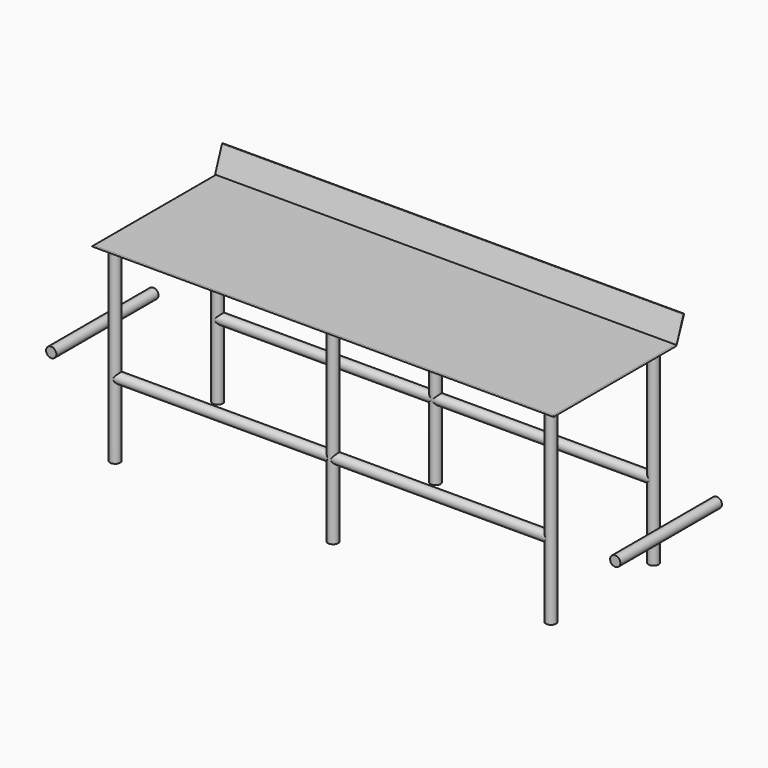
from build123d import *

# Parameters (mm, degrees)
F0_R        = 20
F1_DEPTH    = 740
F2_W        = 1800
F2_H        = 600
F3_DEPTH    = 3
F5_DEPTH    = 1800
F6_T1_DEPTH = 623.1732604525
F6_T3_DEPTH = 1823.1732604525
F8_R        = 20
F9_DEPTH    = 1696.72
F11_R       = 20
F12_DEPTH   = 495.3
F14_R       = 20
F15_DEPTH   = 1696.72
F17_R       = 20
F18_DEPTH   = 497.84


# Not quite as in the source:
# - a fillet or chamfer that OpenCascade refuses, or shapes differently, is made with other operations: its cross-section is extruded or revolved along the edge and cut away or added


with BuildPart() as f1:
    # F0 (on Top) → F1 (new body)
    with BuildSketch(Plane.XY):
        with Locations((-850, 250)):
            Circle(F0_R)
    extrude(amount=F1_DEPTH)


with BuildPart() as f1b:
    # F0 (on Top) → F1, piece 2 (new body)
    with BuildSketch(Plane.XY):
        with Locations((-850, -250)):
            Circle(F0_R)
    extrude(amount=F1_DEPTH)


with BuildPart() as f1c:
    # F0 (on Top) → F1, piece 3 (new body)
    with BuildSketch(Plane.XY):
        with Locations((850, 250)):
            Circle(F0_R)
    extrude(amount=F1_DEPTH)

    # F14 (on face) → F15 (join)
    with BuildSketch(Plane.YZ.offset(850)):
        with Locations((249.8890012503, 290)):
            Circle(F14_R)
    extrude(amount=-F15_DEPTH)


with BuildPart() as f1d:
    # F0 (on Top) → F1, piece 4 (new body)
    with BuildSketch(Plane.XY):
        with Locations((850, -250)):
            Circle(F0_R)
    extrude(amount=F1_DEPTH)


with BuildPart() as f1e:
    # F0 (on Top) → F1, piece 5 (new body)
    with BuildSketch(Plane.XY):
        with Locations((0, 250)):
            Circle(F0_R)
    extrude(amount=F1_DEPTH)


with BuildPart() as f1f:
    # F0 (on Top) → F1, piece 6 (new body)
    with BuildSketch(Plane.XY):
        with Locations((0, -250)):
            Circle(F0_R)
    extrude(amount=F1_DEPTH)


with BuildPart() as f3:
    # F2 (on face) → F3 (new body)
    with BuildSketch(Plane.XY.offset(740)):
        Rectangle(F2_W, F2_H)
    extrude(amount=F3_DEPTH)

    # F6: fillet of radius 5.08 on 3 edges, made by hand

    # F6_s2 → F6_t1 (cut)
    with BuildSketch(Plane.XZ.offset(-311.5866302263)):
        with BuildLine():
            ThreePointArc((900, 740), (898.1257826579, 742.1845515591), (895.3653479095, 743))
            Line((895.3653479095, 743), (900, 743))
            Line((900, 743), (900, 740))
        make_face()
        with BuildLine():
            ThreePointArc((-900, 740), (-898.1257826579, 742.1845515591), (-895.3653479095, 743))
            Line((-895.3653479095, 743), (-900, 743))
            Line((-900, 743), (-900, 740))
        make_face()
    extrude(amount=F6_T1_DEPTH, mode=Mode.SUBTRACT)

    # F6_s4 → F6_t3 (cut)
    with BuildSketch(Plane.YZ.offset(-911.5866302263)):
        with BuildLine():
            ThreePointArc((-300, 740), (-298.1257826579, 742.1845515591), (-295.3653479095, 743))
            Line((-295.3653479095, 743), (-300, 743))
            Line((-300, 743), (-300, 740))
        make_face()
    extrude(amount=F6_T3_DEPTH, mode=Mode.SUBTRACT)


with BuildPart() as f5:
    # F4 (on face) → F5 (new body, through all)
    with BuildSketch(Plane(origin=(-900, 0, 0), x_dir=(0, -1, 0), z_dir=(-1, 0, 0))):
        with BuildLine():
            Line((-336.2584676847, 834.0285967724), (-300, 743))
            Line((-300, 743), (-333.5179740459, 835.089876837))
            ThreePointArc((-333.5179740459, 835.089876837), (-334.3171677089, 836.089043654), (-335.5584418841, 836.3993390954))
            ThreePointArc((-335.5584418841, 836.3993390954), (-336.3185674809, 835.3350648013), (-336.2584676847, 834.0285967724))
        make_face()
    extrude(amount=-F5_DEPTH)


with BuildPart() as f5b:
    # F4 (on face) → F5, piece 2 (new body, through all)
    with BuildSketch(Plane(origin=(-900, 0, 0), x_dir=(0, -1, 0), z_dir=(-1, 0, 0))):
        with BuildLine():
            ThreePointArc((-336.0813995741, 836.2852217919), (-335.8237556544, 836.3598544977), (-335.5584418841, 836.3993390954))
            ThreePointArc((-335.5584418841, 836.3993390954), (-335.3298195345, 836.5396325429), (-335.0844798629, 836.6480708928))
            Line((-335.0844798629, 836.6480708928), (-336.0813995741, 836.2852217919))
        make_face()
    extrude(amount=-F5_DEPTH)


with BuildPart() as f9:
    # F8 (on face) → F9 (new body)
    with BuildSketch(Plane.YZ.offset(-850)):
        with Locations((-249.004855752, 290)):
            Circle(F8_R)
    extrude(amount=F9_DEPTH)


with BuildPart() as f12:
    # F11 (on face) → F12 (new body)
    with BuildSketch(Plane(origin=(0, -250, 0), x_dir=(-1, 0, 0), z_dir=(0, 1, 0))):
        with Locations((-1100.4728078842, 290)):
            Circle(F11_R)
    extrude(amount=F12_DEPTH)


with BuildPart() as f18:
    # F17 (on face) → F18 (new body)
    with BuildSketch(Plane(origin=(0, 250, 0), x_dir=(-1, 0, 0), z_dir=(0, 1, 0))):
        with Locations((1100.9551286697, 290)):
            Circle(F17_R)
    extrude(amount=-F18_DEPTH)


solid = Compound([f1.part, f1b.part, f1c.part, f1d.part, f1e.part, f1f.part, f3.part, f5.part, f5b.part, f9.part, f12.part, f18.part])
